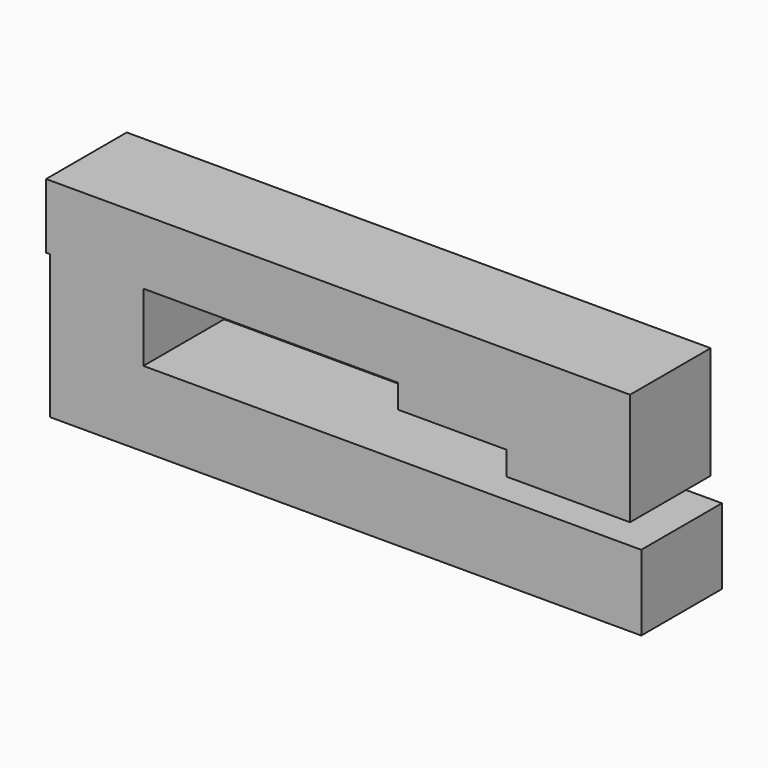
from build123d import *

# Parameters (mm, degrees)
F0_W     = 23.5785879195
F0_H     = 17.130497843
F0_W_2   = 27.351161465
F0_H_2   = 5.9732412919
F1_DEPTH = 25.4


with BuildPart() as f1:
    # F0 (on Front) → F1 (new body)
    with BuildSketch(Plane.XZ):
        Polygon((-47.9431264102, 0), (-71.5217143297, 0), (-71.5217143297, -19.0233327448), (77.4949491024, -19.0233327448), (77.4949491024, 0), align=None)
        with Locations((-59.73242037, 8.5652489215)):
            Rectangle(F0_W, F0_H)
        Polygon((74.6655240655, 5.1840152591), (74.6655240655, 17.130497843), (43.5417890549, 17.130497843), (43.5417890549, 11.1572565511), (43.5417890549, 5.1840152591), align=None)
        with Locations((29.8662083223, 14.1438771971)):
            Rectangle(F0_W_2, F0_H_2)
        Polygon((-72.4648535252, 33.4783159196), (-72.4648535252, 17.130497843), (-71.5217143297, 17.130497843), (-47.9431264102, 17.130497843), (16.1906275898, 17.130497843), (43.5417890549, 17.130497843), (74.6655240655, 17.130497843), (74.6655240655, 33.4783159196), align=None)
    extrude(amount=F1_DEPTH)


solid = f1.part
